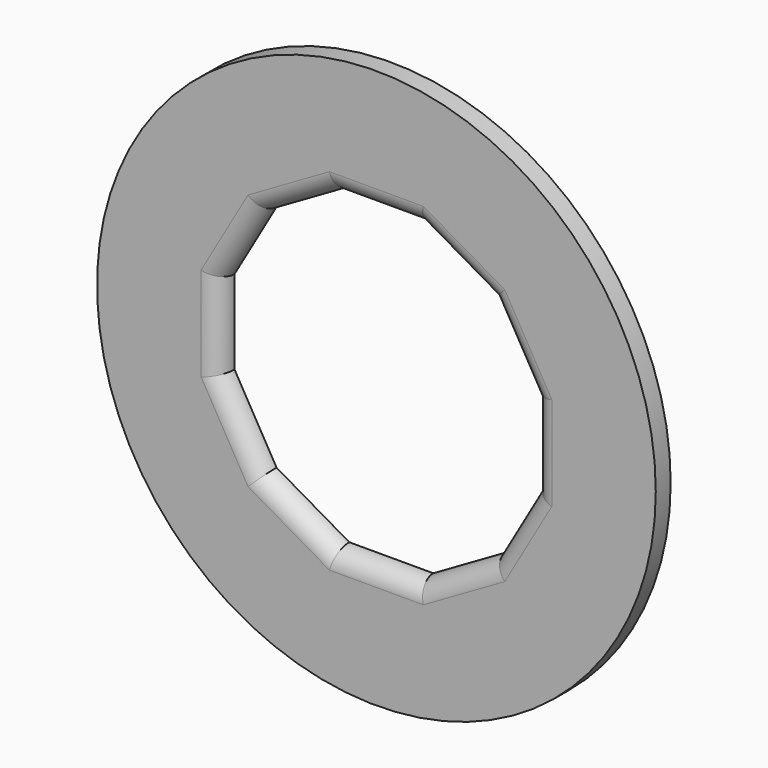
from build123d import *

# Parameters (mm, degrees)
F0_R     = 45
F1_DEPTH = 3
F2_R     = 2.99999


# Not quite as in the source:
# - a fillet or chamfer is up to 0.001 mm smaller than in the source, because OpenCascade refuses the exact size


with BuildPart() as f1:
    # F0 (on Front) → F1 (new body)
    with BuildSketch(Plane.XZ):
        Circle(F0_R)
        Polygon((-18.4842828911, 18.4842828911), (-6.7657171089, 25.25), (6.7657171089, 25.25), (18.4842828911, 18.4842828911), (25.25, 6.7657171089), (25.25, -6.7657171089), (18.4842828911, -18.4842828911), (6.7657171089, -25.25), (-6.7657171089, -25.25), (-18.4842828911, -18.4842828911), (-25.25, -6.7657171089), (-25.25, 6.7657171089), align=None, mode=Mode.SUBTRACT)
    extrude(amount=F1_DEPTH)

    # F2 (radius 3 in the source; OpenCascade refuses exactly that, so slightly less here)
    f2_edges = [f1.edges().sort_by_distance(p)[0] for p in [
        (-12.625, -3, 21.867141),
        (-21.867141, -3, 12.625),
        (-25.25, -3, 0),
        (-21.867141, -3, -12.625),
        (-12.625, -3, -21.867141),
        (0, -3, -25.25),
        (12.625, -3, -21.867141),
        (21.867141, -3, -12.625),
        (25.25, -3, 0),
        (21.867141, -3, 12.625),
        (12.625, -3, 21.867141),
        (0, -3, 25.25),
    ]]
    fillet(f2_edges, radius=F2_R)


solid = f1.part
